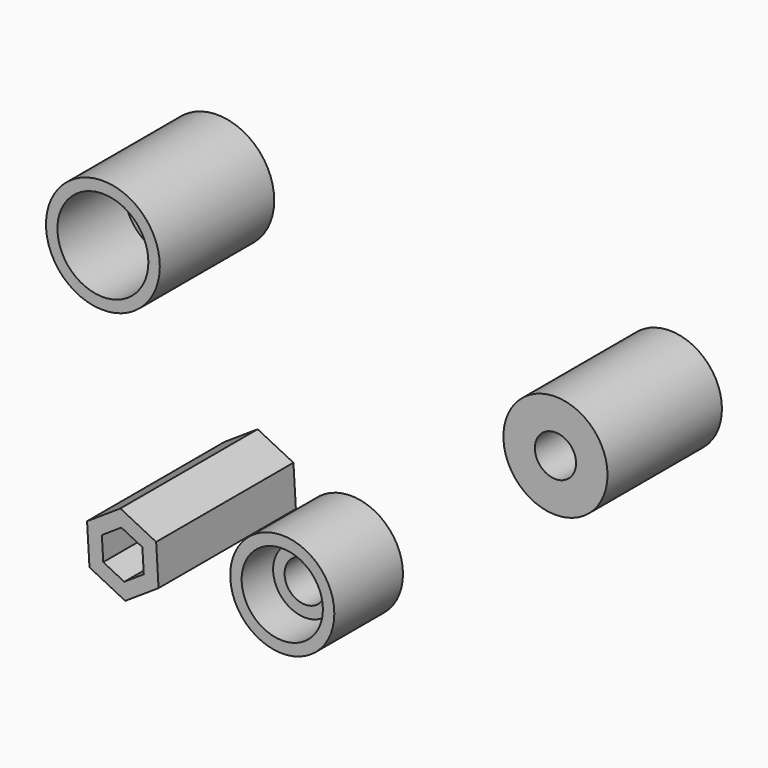
from build123d import *

# Parameters (mm, degrees)
F1_DEPTH  = 30
F2_DEPTH  = 10
F3_R      = 5.6
F3_R_2    = 3.6
F4_DEPTH  = 10
F5_R      = 9.1
F5_R_2    = 7.1
F6_DEPTH  = 15
F7_R      = 9.1
F7_R_2    = 7.1
F7_R_3    = 3.6
F8_DEPTH  = 25
F9_R      = 7.1
F9_R_2    = 3.6
F10_DEPTH = 11.2
F11_R     = 9.95
F11_R_2   = 7.95
F12_DEPTH = 25
F13_R     = 8.00000038
F13_R_2   = 7.1
F14_DEPTH = 10.4


# Not quite as in the source:
# - a feature of the source that left no trace in its solid (it failed there, or was rolled back) is left out


with BuildPart() as f1:
    # F0 (on Front) → F1 (new body)
    with BuildSketch(Plane.XZ):
        Polygon((-22.125422674, 10.1726256458), (-21.6995270296, 3.1996817744), (-15.4478326757, 0.0820462861), (-9.622033966, 3.9373546692), (-10.0479296104, 10.9102985405), (-16.2996239644, 14.0279340289), align=None)
        Polygon((-12.4552844491, 9.3171959029), (-12.2053787404, 5.2256337966), (-15.6238226113, 2.9634280511), (-19.2921721909, 4.7927844121), (-19.5420778996, 8.8843465184), (-16.1236340287, 11.1465522638), align=None, mode=Mode.SUBTRACT)
    extrude(amount=F1_DEPTH)

    # F0 (on Front) → F2 (join)
    with BuildSketch(Plane.XZ):
        Polygon((-15.6238226113, 2.9634280511), (-12.2053787404, 5.2256337966), (-12.4552844491, 9.3171959029), (-16.1236340287, 11.1465522638), (-19.5420778996, 8.8843465184), (-19.2921721909, 4.7927844121), align=None)
    extrude(amount=F2_DEPTH)


with BuildPart() as f4:
    # F3 (on Front) → F4 (new body)
    with BuildSketch(Plane.XZ):
        Circle(F3_R)
        Circle(F3_R_2, mode=Mode.SUBTRACT)
    extrude(amount=F4_DEPTH)


with BuildPart() as f6:
    # F5 (on Front) → F6 (new body)
    with BuildSketch(Plane.XZ):
        Circle(F5_R)
        Circle(F5_R_2, mode=Mode.SUBTRACT)
    extrude(amount=F6_DEPTH)


with BuildPart() as f8:
    # F7 (on Front) → F8 (new body)
    with BuildSketch(Plane.XZ):
        with Locations((55.7573027909, 43.5424260795)):
            Circle(F7_R)
        with Locations((55.7573027909, 43.5424260795)):
            Circle(F7_R_2, mode=Mode.SUBTRACT)
        with Locations((55.7573027909, 43.5424260795)):
            Circle(F7_R_2)
        with Locations((55.7573027909, 43.5424260795)):
            Circle(F7_R_3, mode=Mode.SUBTRACT)
    extrude(amount=F8_DEPTH)

    # F9 (on face) → F10 (cut)
    with BuildSketch(Plane(origin=(0, 0, 0), x_dir=(-1, 0, 0), z_dir=(0, 1, 0))):
        with Locations((-55.7573027909, 43.5424260795)):
            Circle(F9_R)
        with Locations((-55.7573027909, 43.5424260795)):
            Circle(F9_R_2, mode=Mode.SUBTRACT)
    extrude(amount=-F10_DEPTH, mode=Mode.SUBTRACT)


with BuildPart() as f12:
    # F11 (on Front) → F12 (new body)
    with BuildSketch(Plane.XZ):
        with Locations((-23.3567170799, 50.1853749156)):
            Circle(F11_R)
        with Locations((-23.3567170799, 50.1853749156)):
            Circle(F11_R_2, mode=Mode.SUBTRACT)
    extrude(amount=F12_DEPTH)

    # F13 (on face) → F14 (join)
    with BuildSketch(Plane(origin=(0, 0, 0), x_dir=(-1, 0, 0), z_dir=(0, 1, 0))):
        with Locations((23.3567170799, 50.1853749156)):
            Circle(F13_R)
        with Locations((23.3567170799, 50.1853749156)):
            Circle(F13_R_2, mode=Mode.SUBTRACT)
    extrude(amount=-F14_DEPTH)


solid = Compound([f1.part, f4.part, f6.part, f8.part, f12.part])
